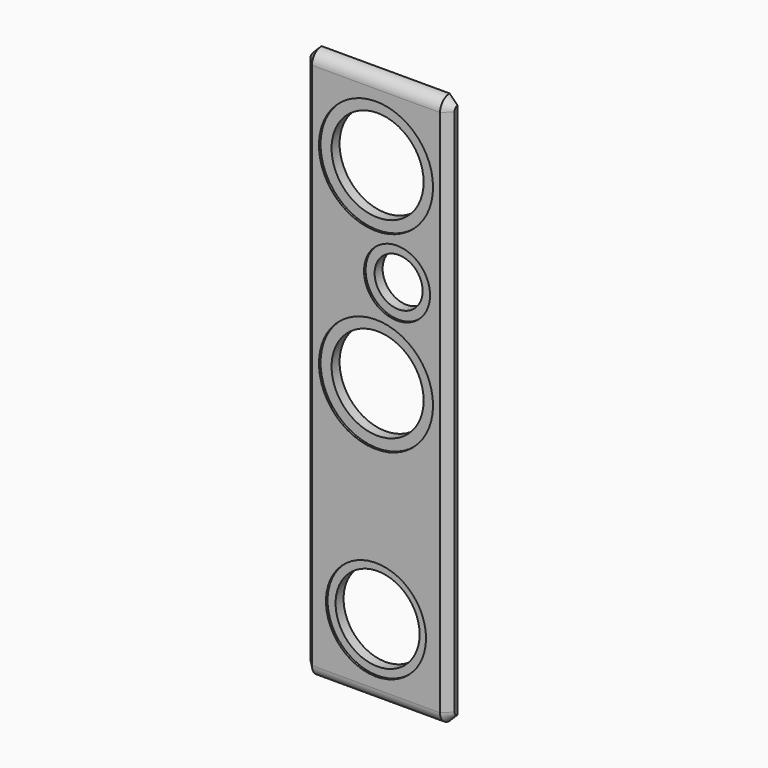
from build123d import *

# Parameters (mm, degrees)
F0_W         = 228.6
F0_H         = 876.3
F0_R         = 79.375
F0_R_2       = 90.4875
F0_R_3       = 52.3875
F0_R_4       = 73.025
F0_R_5       = 38.1
F0_R_6       = 66.675
F1_DEPTH     = 19.05
F2_DEPTH     = 3.175
F4_R         = 19.04999
F5_T1_DEPTH  = 838.20002
F5_T3_DEPTH  = 32.6603839472
F5_T6_ANGLE  = 90
F5_T8_ANGLE  = 90
F5_T10_ANGLE = 90
F5_T12_ANGLE = 90


# Not quite as in the source:
# - a fillet or chamfer that OpenCascade refuses, or shapes differently, is made with other operations: its cross-section is extruded or revolved along the edge and cut away or added
# - a fillet or chamfer is up to 0.001 mm smaller than in the source, because OpenCascade refuses the exact size


with BuildPart() as f1:
    # F0 (on Front) → F1 (new body)
    with BuildSketch(Plane.XZ):
        with Locations((0, 476.25)):
            Rectangle(F0_W, F0_H)
        with Locations((0, 153.9875)):
            Circle(F0_R, mode=Mode.SUBTRACT)
        with Locations((0, 482.6)):
            Circle(F0_R_2, mode=Mode.SUBTRACT)
        with Locations((33.3502, 635)):
            Circle(F0_R_3, mode=Mode.SUBTRACT)
        with Locations((0, 787.4)):
            Circle(F0_R_2, mode=Mode.SUBTRACT)
        with Locations((0, 787.4)):
            Circle(F0_R_2)
        with Locations((0, 787.4)):
            Circle(F0_R_4, mode=Mode.SUBTRACT)
        with Locations((33.3502, 635)):
            Circle(F0_R_3)
        with Locations((33.3502, 635)):
            Circle(F0_R_5, mode=Mode.SUBTRACT)
        with Locations((0, 482.6)):
            Circle(F0_R_2)
        with Locations((0, 482.6)):
            Circle(F0_R_4, mode=Mode.SUBTRACT)
        with Locations((0, 153.9875)):
            Circle(F0_R)
        with Locations((0, 153.9875)):
            Circle(F0_R_6, mode=Mode.SUBTRACT)
    extrude(amount=-F1_DEPTH)

    # F0 (on Front) → F2 (cut)
    with BuildSketch(Plane.XZ):
        with Locations((0, 787.4)):
            Circle(F0_R_2)
        with Locations((0, 787.4)):
            Circle(F0_R_4, mode=Mode.SUBTRACT)
        with Locations((33.3502, 635)):
            Circle(F0_R_3)
        with Locations((33.3502, 635)):
            Circle(F0_R_5, mode=Mode.SUBTRACT)
        with Locations((0, 482.6)):
            Circle(F0_R_2)
        with Locations((0, 482.6)):
            Circle(F0_R_4, mode=Mode.SUBTRACT)
        with Locations((0, 153.9875)):
            Circle(F0_R)
        with Locations((0, 153.9875)):
            Circle(F0_R_6, mode=Mode.SUBTRACT)
    extrude(amount=-F2_DEPTH, mode=Mode.SUBTRACT)

    # F4 (radius 19.05 in the source; OpenCascade refuses exactly that, so slightly less here)
    f4_edges = [f1.edges().sort_by_distance(p)[0] for p in [
        (0, 0, 914.4),
        (0, 0, 38.1),
    ]]
    fillet(f4_edges, radius=F4_R)

    # F5: chamfer of 12.7 on 2 edges, made by hand

    # F5_s2 → F5_t1 (cut)
    with BuildSketch(Plane.XY.offset(57.14999)):
        Polygon((-101.6, 0), (-114.3, 12.7), (-114.3, 0), align=None)
        Polygon((114.3, 12.7), (101.6, 0), (114.3, 0), align=None)
    extrude(amount=F5_T1_DEPTH, mode=Mode.SUBTRACT)

    # F5_s4 → F5_t3 (cut)
    with BuildSketch(Plane.XZ.offset(-51.7103739472)):
        Polygon((114.3, 901.7), (101.6, 914.4), (114.3, 914.4), align=None)
        Polygon((114.3, 50.8), (101.6, 38.1), (114.3, 38.1), align=None)
        Polygon((-101.6, 38.1), (-114.3, 50.8), (-114.3, 38.1), align=None)
        Polygon((-101.6, 914.4), (-114.3, 901.7), (-114.3, 914.4), align=None)
    extrude(amount=F5_T3_DEPTH, mode=Mode.SUBTRACT)

    # F5_s5 → F5_t6 (revolve, cut)
    with BuildSketch(Plane.XZ.offset(-19.04999)):
        Polygon((114.3, 50.8), (101.6, 38.1), (114.3, 38.1), align=None)
    revolve(axis=Axis((114.3, 19.04999, 57.14999), (-1, 0, 0)), revolution_arc=F5_T6_ANGLE, mode=Mode.SUBTRACT)

    # F5_s7 → F5_t8 (revolve, cut)
    with BuildSketch(Plane.XZ.offset(-19.04999)):
        Polygon((114.3, 901.7), (101.6, 914.4), (114.3, 914.4), align=None)
    revolve(axis=Axis((114.3, 19.04999, 895.35001), (1, 0, 0)), revolution_arc=F5_T8_ANGLE, mode=Mode.SUBTRACT)

    # F5_s9 → F5_t10 (revolve, cut)
    with BuildSketch(Plane.XZ.offset(-19.04999)):
        Polygon((-101.6, 914.4), (-114.3, 901.7), (-114.3, 914.4), align=None)
    revolve(axis=Axis((-114.3, 19.04999, 895.35001), (1, 0, 0)), revolution_arc=F5_T10_ANGLE, mode=Mode.SUBTRACT)

    # F5_s11 → F5_t12 (revolve, cut)
    with BuildSketch(Plane.XZ.offset(-19.04999)):
        Polygon((-101.6, 38.1), (-114.3, 50.8), (-114.3, 38.1), align=None)
    revolve(axis=Axis((-114.3, 19.04999, 57.14999), (-1, 0, 0)), revolution_arc=F5_T12_ANGLE, mode=Mode.SUBTRACT)


solid = f1.part
